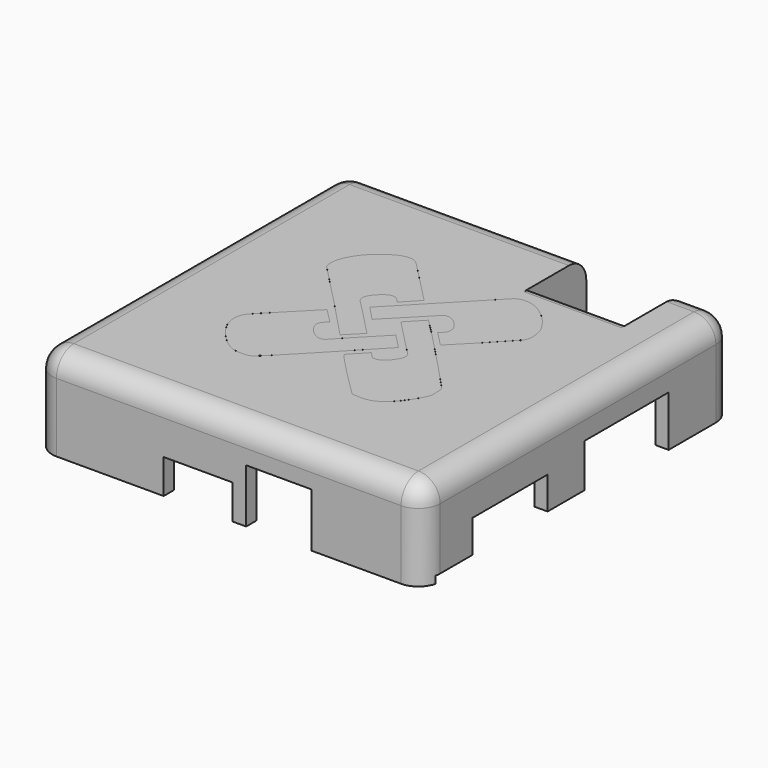
from build123d import *

# Parameters (mm, degrees)
F0_W          = 50
F0_H          = 50
F0_R          = 2.375
F1_DEPTH      = 1.5
F0_R_2        = 1.25
F2_DEPTH      = 8
F2_DEPTH_BACK = 1.5
F0_W_2        = 53.6
F0_H_2        = 53.6
F3_DEPTH      = 11
F3_DEPTH_BACK = 1.5
F4_W          = 9.5
F4_H          = 2
F4_H_2        = 2.75
F4_W_2        = 9
F4_H_3        = 2.25
F4_H_4        = 5.2
F5_DEPTH      = 26.801
F6_W          = 5.25
F6_H          = 1.1261866987
F6_W_2        = 1.14
F6_W_3        = 13
F6_H_2        = 1.5
F6_W_4        = 14.5
F6_H_3        = 6
F6_W_5        = 6.25
F6_H_4        = 3
F7_DEPTH      = 26.801
F9_W          = 9.3
F9_H          = 1.5
F9_W_2        = 1.2
F10_DEPTH     = 13.5
F11_DEPTH     = 13.5
F12_DEPTH     = 1.2
F13_T1_DEPTH  = 11.3
F13_T3_DEPTH  = 37.8
F13_T5_DEPTH  = 47.6
F13_T7_DEPTH  = 47.6
F13_T9_DEPTH  = 17
F13_T11_DEPTH = 18
F13_S15_W     = 3.06
F13_S15_H     = 3.06
F13_T16_DEPTH = 3.06
F13_S21_W     = 3.06
F13_S21_H     = 3.06
F13_T22_DEPTH = 3.06
F13_S27_W     = 3.06
F13_S27_H     = 3.06
F13_T28_DEPTH = 3.06
F13_S33_W     = 3.06
F13_S33_H     = 3.06
F13_T34_DEPTH = 3.06
F14_R         = 1.5
F15_W         = 14
F15_H         = 2
F16_DEPTH     = 26.801
F18_DEPTH     = 1.501
F19_DEPTH     = 1.5


# Not quite as in the source:
# - a fillet or chamfer that OpenCascade refuses, or shapes differently, is made with other operations: its cross-section is extruded or revolved along the edge and cut away or added


with BuildPart() as f1:
    # F0 (on Top) → F1 (new body)
    with BuildSketch(Plane.XY):
        Rectangle(F0_W, F0_H)
        with Locations((-21.5, -22)):
            Circle(F0_R, mode=Mode.SUBTRACT)
        with Locations((21.5, -22)):
            Circle(F0_R, mode=Mode.SUBTRACT)
        with Locations((-21.5, 22)):
            Circle(F0_R, mode=Mode.SUBTRACT)
        with Locations((22.25, 22)):
            Circle(F0_R, mode=Mode.SUBTRACT)
    extrude(amount=F1_DEPTH)



with BuildPart() as f1b:
    # F0 (on Top) → F1, piece 2 (new body)
    with BuildSketch(Plane.XY):
        with Locations((-21.5, 22)):
            Circle(F0_R_2)
    extrude(amount=F1_DEPTH)


with BuildPart() as f1c:
    # F0 (on Top) → F1, piece 3 (new body)
    with BuildSketch(Plane.XY):
        with Locations((22.25, 22)):
            Circle(F0_R_2)
    extrude(amount=F1_DEPTH)


with BuildPart() as f1d:
    # F0 (on Top) → F1, piece 4 (new body)
    with BuildSketch(Plane.XY):
        with Locations((21.5, -22)):
            Circle(F0_R_2)
    extrude(amount=F1_DEPTH)


with BuildPart() as f1e:
    # F0 (on Top) → F1, piece 5 (new body)
    with BuildSketch(Plane.XY):
        with Locations((-21.5, -22)):
            Circle(F0_R_2)
    extrude(amount=F1_DEPTH)


with BuildPart() as f1_1:
    add(f1.part)

    add(f1b.part)  # F2 merges F1b

    add(f1c.part)  # F2 merges F1c

    add(f1d.part)  # F2 merges F1d

    add(f1e.part)  # F2 merges F1e
    # F0 (on Top) → F2 (join, two sides)
    with BuildSketch(Plane.XY) as f2_sk:
        with Locations((-21.5, 22)):
            Circle(F0_R)
        with Locations((-21.5, 22)):
            Circle(F0_R_2, mode=Mode.SUBTRACT)
        with Locations((22.25, 22)):
            Circle(F0_R)
        with Locations((22.25, 22)):
            Circle(F0_R_2, mode=Mode.SUBTRACT)
        with Locations((21.5, -22)):
            Circle(F0_R)
        with Locations((21.5, -22)):
            Circle(F0_R_2, mode=Mode.SUBTRACT)
        with Locations((-21.5, -22)):
            Circle(F0_R)
        with Locations((-21.5, -22)):
            Circle(F0_R_2, mode=Mode.SUBTRACT)
    extrude(amount=-F2_DEPTH)
    extrude(f2_sk.sketch, amount=F2_DEPTH_BACK)

    # F0 (on Top) → F3 (join, two sides)
    with BuildSketch(Plane.XY) as f3_sk:
        Rectangle(F0_W_2, F0_H_2)
        Rectangle(F0_W, F0_H, mode=Mode.SUBTRACT)
    extrude(amount=-F3_DEPTH)
    extrude(f3_sk.sketch, amount=F3_DEPTH_BACK)

    # F4 (on Front) → F5 (cut, through all)
    with BuildSketch(Plane.XZ):
        with Locations((-4.25, -7.25)):
            Rectangle(F4_W, F4_H)
        with Locations((-4.25, -9.625)):
            Rectangle(F4_W, F4_H_2)
        with Locations((6.9, -9.875)):
            Rectangle(F4_W_2, F4_H_3)
        with Locations((6.9, -6.15)):
            Rectangle(F4_W_2, F4_H_4)
    extrude(amount=F5_DEPTH, mode=Mode.SUBTRACT)

    # F6 (on Right) → F7 (cut, through all)
    with BuildSketch(Plane.YZ):
        with Locations((-2.625, -10.5630933493)):
            Rectangle(F6_W, F6_H)
        with Locations((0.57, -10.5630933493)):
            Rectangle(F6_W_2, F6_H)
        with Locations((-11.75, -10.5630933493)):
            Rectangle(F6_W_3, F6_H)
        with Locations((-11.75, -9.25)):
            Rectangle(F6_W_3, F6_H_2)
        with Locations((8.39, -7)):
            Rectangle(F6_W_4, F6_H_3)
        with Locations((8.39, -10.5630933493)):
            Rectangle(F6_W_4, F6_H)
        with Locations((-21.375, -10.5630933493)):
            Rectangle(F6_W_5, F6_H)
        with Locations((-11.75, -7)):
            Rectangle(F6_W_3, F6_H_4)
    extrude(amount=F7_DEPTH, mode=Mode.SUBTRACT)

    # F9 (on offset) → F10 (cut)
    with BuildSketch(Plane.YZ.offset(6.5)):
        Polygon((26.8, -9), (26.8, 0), (17.5, 0), (17.5, -5.8), (17.5, -9), align=None)
        with Locations((22.15, 0.75)):
            Rectangle(F9_W, F9_H)
        Polygon((17.5, -5.8), (17.5, 0), (16.3, 0), (16.3, -9), (17.5, -9), align=None)
        with Locations((16.9, 0.75)):
            Rectangle(F9_W_2, F9_H)
    extrude(amount=F10_DEPTH, mode=Mode.SUBTRACT)

    # F9 (on offset) → F11 (join)
    with BuildSketch(Plane.YZ.offset(6.5)):
        Polygon((17.5, -5.8), (17.5, 0), (16.3, 0), (16.3, -9), (17.5, -9), align=None)
        with Locations((16.9, 0.75)):
            Rectangle(F9_W_2, F9_H)
    extrude(amount=F11_DEPTH)

    # F9 (on offset) → F12 (join)
    with BuildSketch(Plane.YZ.offset(6.5)):
        Polygon((26.8, -9), (26.8, 0), (17.5, 0), (17.5, -5.8), (17.5, -9), align=None)
        with Locations((22.15, 0.75)):
            Rectangle(F9_W, F9_H)
        Polygon((17.5, -5.8), (17.5, 0), (16.3, 0), (16.3, -9), (17.5, -9), align=None)
        with Locations((16.9, 0.75)):
            Rectangle(F9_W_2, F9_H)
    extrude(amount=-F12_DEPTH)

    # F13: fillet of radius 3 on 10 edges, made by hand

    # F13_s2 → F13_t1 (cut)
    with BuildSketch(Plane.YZ.offset(12.5)):
        with BuildLine():
            ThreePointArc((23.8, 1.5), (25.9213203436, 0.6213203436), (26.8, -1.5))
            Line((26.8, -1.5), (26.8, 1.5))
            Line((26.8, 1.5), (23.8, 1.5))
        make_face()
    extrude(amount=F13_T1_DEPTH, mode=Mode.SUBTRACT)

    # F13_s4 → F13_t3 (cut)
    with BuildSketch(Plane.YZ.offset(-23.8)):
        with BuildLine():
            ThreePointArc((23.8, 1.5), (25.9213203436, 0.6213203436), (26.8, -1.5))
            Line((26.8, -1.5), (26.8, 1.5))
            Line((26.8, 1.5), (23.8, 1.5))
        make_face()
    extrude(amount=F13_T3_DEPTH, mode=Mode.SUBTRACT)

    # F13_s6 → F13_t5 (cut)
    with BuildSketch(Plane.XZ.offset(-23.8)):
        with BuildLine():
            ThreePointArc((-23.8, 1.5), (-25.9213203436, 0.6213203436), (-26.8, -1.5))
            Line((-26.8, -1.5), (-26.8, 1.5))
            Line((-26.8, 1.5), (-23.8, 1.5))
        make_face()
        with BuildLine():
            ThreePointArc((23.8, 1.5), (25.9213203436, 0.6213203436), (26.8, -1.5))
            Line((26.8, -1.5), (26.8, 1.5))
            Line((26.8, 1.5), (23.8, 1.5))
        make_face()
    extrude(amount=F13_T5_DEPTH, mode=Mode.SUBTRACT)

    # F13_s8 → F13_t7 (cut)
    with BuildSketch(Plane.YZ.offset(-23.8)):
        with BuildLine():
            ThreePointArc((-23.8, 1.5), (-25.9213203436, 0.6213203436), (-26.8, -1.5))
            Line((-26.8, -1.5), (-26.8, 1.5))
            Line((-26.8, 1.5), (-23.8, 1.5))
        make_face()
    extrude(amount=F13_T7_DEPTH, mode=Mode.SUBTRACT)

    # F13_s10 → F13_t9 (cut)
    with BuildSketch(Plane.XY.offset(-18.5)):
        with BuildLine():
            ThreePointArc((-26.8, -23.8), (-25.9213203436, -25.9213203436), (-23.8, -26.8))
            Line((-23.8, -26.8), (-26.8, -26.8))
            Line((-26.8, -26.8), (-26.8, -23.8))
        make_face()
        with BuildLine():
            ThreePointArc((23.8, 26.8), (25.9213203436, 25.9213203436), (26.8, 23.8))
            Line((26.8, 23.8), (26.8, 26.8))
            Line((26.8, 26.8), (23.8, 26.8))
        make_face()
        with BuildLine():
            ThreePointArc((26.8, -23.8), (25.9213203436, -25.9213203436), (23.8, -26.8))
            Line((23.8, -26.8), (26.8, -26.8))
            Line((26.8, -26.8), (26.8, -23.8))
        make_face()
        with BuildLine():
            ThreePointArc((-26.8, 23.8), (-25.9213203436, 25.9213203436), (-23.8, 26.8))
            Line((-23.8, 26.8), (-26.8, 26.8))
            Line((-26.8, 26.8), (-26.8, 23.8))
        make_face()
    extrude(amount=F13_T9_DEPTH, mode=Mode.SUBTRACT)

    # F13_s12 → F13_t11 (cut)
    with BuildSketch(Plane.XY.offset(-9)):
        with BuildLine():
            ThreePointArc((23, 26.8), (20.8786796564, 25.9213203436), (20, 23.8))
            Line((20, 23.8), (20, 26.8))
            Line((20, 26.8), (23, 26.8))
        make_face()
    extrude(amount=F13_T11_DEPTH, mode=Mode.SUBTRACT)


with BuildPart() as f13_tool14:
    # F13_s15 → F13_t16 (new body)
    with BuildSketch(Plane.XY.offset(-1.5)):
        with Locations((25.33, 25.33)):
            Rectangle(F13_S15_W, F13_S15_H)
    extrude(amount=F13_T16_DEPTH)

    # F13_s17 → F13_t18 (revolve, cut)
    with BuildSketch(Plane(origin=(23.8, 23.8, -1.5), x_dir=(-0.7071067812, -0.7071067812, 0), z_dir=(-0.7071067812, 0.7071067812, 0))):
        with BuildLine():
            ThreePointArc((0, -3), (3, 0), (0, 3))
            Line((0, 3), (0, -3))
        make_face()
    revolve(axis=Axis((23.8, 23.8, -1.5), (0, 0, 1)), mode=Mode.SUBTRACT)


with BuildPart() as f1_2:
    add(f1_1.part)

    # F13_t13: cut F13_tool14
    add(f13_tool14.part, mode=Mode.SUBTRACT)


with BuildPart() as f13_tool20:
    # F13_s21 → F13_t22 (new body)
    with BuildSketch(Plane.XY.offset(-1.5)):
        with Locations((-25.33, 25.33)):
            Rectangle(F13_S21_W, F13_S21_H)
    extrude(amount=F13_T22_DEPTH)

    # F13_s23 → F13_t24 (revolve, cut)
    with BuildSketch(Plane(origin=(-23.8, 23.8, -1.5), x_dir=(0.7071067812, -0.7071067812, 0), z_dir=(-0.7071067812, -0.7071067812, 0))):
        with BuildLine():
            ThreePointArc((0, -3), (3, 0), (0, 3))
            Line((0, 3), (0, -3))
        make_face()
    revolve(axis=Axis((-23.8, 23.8, -1.5), (0, 0, 1)), mode=Mode.SUBTRACT)


with BuildPart() as f1_3:
    add(f1_2.part)

    # F13_t19: cut F13_tool20
    add(f13_tool20.part, mode=Mode.SUBTRACT)


with BuildPart() as f13_tool26:
    # F13_s27 → F13_t28 (new body)
    with BuildSketch(Plane.XY.offset(-1.5)):
        with Locations((-25.33, -25.33)):
            Rectangle(F13_S27_W, F13_S27_H)
    extrude(amount=F13_T28_DEPTH)

    # F13_s29 → F13_t30 (revolve, cut)
    with BuildSketch(Plane(origin=(-23.8, -23.8, -1.5), x_dir=(0.7071067812, 0.7071067812, 0), z_dir=(0.7071067812, -0.7071067812, 0))):
        with BuildLine():
            ThreePointArc((0, -3), (3, 0), (0, 3))
            Line((0, 3), (0, -3))
        make_face()
    revolve(axis=Axis((-23.8, -23.8, -1.5), (0, 0, 1)), mode=Mode.SUBTRACT)


with BuildPart() as f1_4:
    add(f1_3.part)

    # F13_t25: cut F13_tool26
    add(f13_tool26.part, mode=Mode.SUBTRACT)


with BuildPart() as f13_tool32:
    # F13_s33 → F13_t34 (new body)
    with BuildSketch(Plane.XY.offset(-1.5)):
        with Locations((25.33, -25.33)):
            Rectangle(F13_S33_W, F13_S33_H)
    extrude(amount=F13_T34_DEPTH)

    # F13_s35 → F13_t36 (revolve, cut)
    with BuildSketch(Plane(origin=(23.8, -23.8, -1.5), x_dir=(-0.7071067812, 0.7071067812, 0), z_dir=(0.7071067812, 0.7071067812, 0))):
        with BuildLine():
            ThreePointArc((0, -3), (3, 0), (0, 3))
            Line((0, 3), (0, -3))
        make_face()
    revolve(axis=Axis((23.8, -23.8, -1.5), (0, 0, 1)), mode=Mode.SUBTRACT)


with BuildPart() as f1_5:
    add(f1_4.part)

    # F13_t31: cut F13_tool32
    add(f13_tool32.part, mode=Mode.SUBTRACT)

    # F14
    f14_edges = [f1_5.edges().sort_by_distance(p)[0] for p in [
        (13.25, 17.5, 1.5),
    ]]
    fillet(f14_edges, radius=F14_R)

    # F15 (on Right) → F16 (cut, through all)
    with BuildSketch(Plane.YZ):
        with Locations((5.75, -7)):
            Rectangle(F15_W, F15_H)
        Polygon((0, -9), (12.75, -9), (12.75, -8), (-1.25, -8), (-1.25, -9), align=None)
        Polygon((-1.25, -10), (12.75, -10), (12.75, -9), (0, -9), (-1.25, -9), align=None)
        Polygon((24.5, -11.0357031226), (24.5, -10), (12.75, -10), (-1.25, -10), (-24.5, -10), (-24.5, -11.0357031226), align=None)
    extrude(amount=-F16_DEPTH, mode=Mode.SUBTRACT)

    # F17 (on Top) → F18 (cut, through all)
    with BuildSketch(Plane.XY):
        with BuildLine():
            add(Edge.make_bspline(
                [(2.6337690446, 4.3777345257), (4.1488296736, 2.9862137615), (13.7044419796, -7.0613876037), (13.5967130417, -7.0670198624), (13.8283273456, -7.3413269189), (13.842337494, -7.82768897), (13.8589220392, -8.8789827644), (13.8432255163, -9.4133274272), (12.1466871073, -12.5160741004), (9.4814131223, -14.6061680167), (7.0123368743, -14.178122061), (6.9283058087, -14.2847187871), (1.0148528171, -8.2934063985), (0.4936719155, -7.5717363434)],
                knots=[0.0089761431, 0.0089761431, 0.0089761431, 0.0089761431, 0.122228571, 0.1330252954, 0.1487734192, 0.1707765281, 0.2013334728, 0.2237533849, 0.2793698301, 0.3371429814, 0.3805089088, 0.3957619618, 0.4879281659, 0.4879281659, 0.4879281659, 0.4879281659], degree=3))
            Line((2.6337690446, 4.3777345257), (0.5629178592, 2.207118169))
            add(Edge.make_bspline(
                [(2.5589191396, -5.4010140019), (2.7372058883, -5.5464348869), (3.2459220871, -6.1241415889), (3.4769231626, -6.2923714077), (4.1870653829, -6.2492504655), (4.5594316814, -6.0075568322), (5.306878931, -5.4483843447), (5.7804633245, -4.6376901998), (5.9797941775, -4.3397540098), (6.0712404556, -3.8231670242), (6.0672996429, -3.3187282043), (5.1979606597, -2.5522554569), (5.2497492592, -2.6206281586), (1.2672758775, 1.4916340736), (0.5629178592, 2.207118169)],
                knots=[0.5848515334, 0.5848515334, 0.5848515334, 0.5848515334, 0.6126188416, 0.63046949, 0.6546842699, 0.6753536997, 0.7048009038, 0.7342593746, 0.752488374, 0.7735556528, 0.7960226968, 0.8266974371, 0.8357204913, 0.9100486613, 0.9100486613, 0.9100486613, 0.9100486613], degree=3))
            Line((2.5589191396, -5.4010140019), (0.4936719155, -7.5717363434))
        make_face()
        with BuildLine():
            add(Edge.make_bspline(
                [(-4.1951583095, 2.7987209668), (1.0080025634, 8.1710432624), (6.5954559155, 13.9403945733), (6.6971467282, 14.0793044814), (7.2582479051, 14.3827174509), (8.0647764726, 14.4893507471), (8.887918878, 14.3534905622), (9.7116687237, 14.0833566665), (10.7682050616, 13.4336081396), (12.09897007, 12.2967113579), (13.0658944102, 10.9673436289), (13.5917626753, 10.0740937493), (13.7533585046, 9.2948130313), (13.8487303283, 8.8038923826), (13.8752502289, 7.8516196297), (13.6781474582, 7.4110605068), (13.5859649447, 7.2050164864)],
                knots=[0.0022926657, 0.0022926657, 0.0022926657, 0.0022926657, 0.2496251328, 0.2701104018, 0.317045917, 0.3751377278, 0.4319642369, 0.4896642967, 0.5591214109, 0.6430144041, 0.7238811151, 0.7877230808, 0.8419106278, 0.8869300511, 0.9471185917, 1, 1, 1, 1], degree=3))
            Line((-4.1951583095, 2.7987209668), (-2.2396288963, 0.7255361531))
            Line((-2.2396288963, 0.7255361531), (3.0672104241, 6.1340472618))
            add(Edge.make_bspline(
                [(3.0672104241, 6.1340472618), (3.143729107, 6.2161982947), (3.297814356, 6.3859570218), (3.6778797918, 6.3840156229), (4.0031329472, 6.3985633539), (4.4692984995, 6.1750311398), (4.8561984925, 5.9176944841), (5.265564945, 5.5805325495), (5.6776892175, 5.0118322743), (6.0193058811, 4.4904086082), (5.9665132612, 3.8963677596), (6.0977186917, 3.5781533203), (5.3779196793, 2.8696377227), (5.2420848817, 2.7216840756)],
                knots=[0, 0, 0, 0, 0.0383458432, 0.0782209102, 0.1166663156, 0.1640685525, 0.2101422145, 0.2587022458, 0.3150733168, 0.3681398035, 0.4175788215, 0.4561043385, 0.5274279887, 0.5274279887, 0.5274279887, 0.5274279887], degree=3))
            Line((5.2420848817, 2.7216840756), (7.2797688511, 0.6421545641))
            add(Edge.make_bspline(
                [(7.2797688511, 0.6421545641), (7.99156258, 1.2587062345), (13.5828543825, 7.1453220507), (13.5822631613, 7.1871017459), (13.5859649447, 7.2050164864)],
                knots=[0.7622871576, 0.7622871576, 0.7622871576, 0.7622871576, 0.9617849206, 0.9820186026, 0.9820186026, 0.9820186026, 0.9820186026], degree=3))
        make_face()
        with BuildLine():
            add(Edge.make_bspline(
                [(-2.6542923727, -4.2488974646), (-2.8543834052, -4.0873226856), (-4.0845557597, -2.6800886543), (-13.7246439358, 7.2979517713), (-13.8311109945, 7.3403793646), (-13.9856307296, 7.981681817), (-13.9110669672, 9.2905656338), (-13.3101549808, 10.628786408), (-12.071793307, 12.3879190858), (-10.1704620865, 13.7773851742), (-8.9247938931, 14.4568163771), (-7.5101780435, 14.5517395208), (-6.8371715752, 14.0554988802), (-6.5565974828, 13.8000496207), (-1.1447687909, 8.2021189611), (-0.6130041743, 7.6959942927)],
                knots=[0.0720940311, 0.0720940311, 0.0720940311, 0.0720940311, 0.1166079175, 0.2264421722, 0.2371589551, 0.2589956261, 0.2931105857, 0.3289547851, 0.3725019507, 0.4179035595, 0.4534919183, 0.4877639959, 0.5119623043, 0.5362346242, 0.6202656763, 0.6202656763, 0.6202656763, 0.6202656763], degree=3))
            Line((-2.6542923727, -4.2488974646), (-0.6209075457, -2.1751756775))
            add(Edge.make_bspline(
                [(-2.62065566, 5.573224122), (-2.63628033, 5.5847033041), (-2.723374723, 5.6744621229), (-3.2713875239, 6.2899087513), (-3.6972074018, 6.4094215205), (-4.3690152372, 6.4131203892), (-5.4810347169, 5.5615218005), (-6.2571863041, 4.4573349954), (-6.2268450742, 3.4853480872), (-5.0025778643, 2.4010071339), (-2.4042081411, -0.3117811964), (-0.6209075457, -2.1751756775)],
                knots=[0.7159990353, 0.7159990353, 0.7159990353, 0.7159990353, 0.7219064655, 0.7491616781, 0.7692248412, 0.7920934858, 0.8269593183, 0.8613429851, 0.8877216064, 0.9231056494, 0.9983359861, 0.9983359861, 0.9983359861, 0.9983359861], degree=3))
            Line((-2.62065566, 5.573224122), (-0.6130041743, 7.6959942927))
        make_face()
        with BuildLine():
            add(Edge.make_bspline(
                [(4.100840015, -2.6277568325), (3.1156892088, -3.6217760081), (-6.7881001653, -14.2180707724), (-7.1441563881, -14.0552668178), (-7.6091691466, -14.2679671408), (-8.3069552716, -14.2284508947), (-9.7962702322, -14.2696213858), (-12.2148557403, -12.3291082124), (-13.9344728603, -9.855657033), (-14.1305245841, -8.0140812071), (-13.7016819828, -6.9022240008), (-13.1236888475, -6.2820192057), (-8.0022842124, -1.0662834705), (-7.4464620694, -0.530619072)],
                knots=[0.0798001793, 0.0798001793, 0.0798001793, 0.0798001793, 0.2014075833, 0.2219962522, 0.2416127947, 0.2672072339, 0.303629489, 0.3577698997, 0.4121374818, 0.4532369288, 0.4838347607, 0.5178463497, 0.6032970918, 0.6032970918, 0.6032970918, 0.6032970918], degree=3))
            Line((4.100840015, -2.6277568325), (2.0720690275, -0.5415278666))
            add(Edge.make_bspline(
                [(-5.4205875749, -2.5717176112), (-5.5411524068, -2.7060819274), (-6.3681922084, -3.4270413154), (-6.1869843049, -4.395556248), (-5.5178214749, -5.3928835237), (-4.6060598952, -6.0525376359), (-3.9678116559, -6.3417089623), (-3.2505155928, -6.148380142), (-2.6634131954, -5.3785788383), (0.0411015742, -2.6151408903), (2.0720690275, -0.5415278666)],
                knots=[0.7094889137, 0.7094889137, 0.7094889137, 0.7094889137, 0.7425186253, 0.7722751956, 0.8061471652, 0.8390403408, 0.8644863284, 0.8888753826, 0.9171555585, 0.9982612727, 0.9982612727, 0.9982612727, 0.9982612727], degree=3))
            Line((-5.4205875749, -2.5717176112), (-7.4464620694, -0.530619072))
        make_face()
    extrude(amount=F18_DEPTH, mode=Mode.SUBTRACT)


with BuildPart() as f19:
    # F17 (on Top) → F19 (new body)
    with BuildSketch(Plane.XY):
        with BuildLine():
            add(Edge.make_bspline(
                [(2.6337690446, 4.3777345257), (4.1488296736, 2.9862137615), (13.7044419796, -7.0613876037), (13.5967130417, -7.0670198624), (13.8283273456, -7.3413269189), (13.842337494, -7.82768897), (13.8589220392, -8.8789827644), (13.8432255163, -9.4133274272), (12.1466871073, -12.5160741004), (9.4814131223, -14.6061680167), (7.0123368743, -14.178122061), (6.9283058087, -14.2847187871), (1.0148528171, -8.2934063985), (0.4936719155, -7.5717363434)],
                knots=[0.0089761431, 0.0089761431, 0.0089761431, 0.0089761431, 0.122228571, 0.1330252954, 0.1487734192, 0.1707765281, 0.2013334728, 0.2237533849, 0.2793698301, 0.3371429814, 0.3805089088, 0.3957619618, 0.4879281659, 0.4879281659, 0.4879281659, 0.4879281659], degree=3))
            Line((2.6337690446, 4.3777345257), (0.5629178592, 2.207118169))
            add(Edge.make_bspline(
                [(2.5589191396, -5.4010140019), (2.7372058883, -5.5464348869), (3.2459220871, -6.1241415889), (3.4769231626, -6.2923714077), (4.1870653829, -6.2492504655), (4.5594316814, -6.0075568322), (5.306878931, -5.4483843447), (5.7804633245, -4.6376901998), (5.9797941775, -4.3397540098), (6.0712404556, -3.8231670242), (6.0672996429, -3.3187282043), (5.1979606597, -2.5522554569), (5.2497492592, -2.6206281586), (1.2672758775, 1.4916340736), (0.5629178592, 2.207118169)],
                knots=[0.5848515334, 0.5848515334, 0.5848515334, 0.5848515334, 0.6126188416, 0.63046949, 0.6546842699, 0.6753536997, 0.7048009038, 0.7342593746, 0.752488374, 0.7735556528, 0.7960226968, 0.8266974371, 0.8357204913, 0.9100486613, 0.9100486613, 0.9100486613, 0.9100486613], degree=3))
            Line((2.5589191396, -5.4010140019), (0.4936719155, -7.5717363434))
        make_face()
    extrude(amount=F19_DEPTH)


with BuildPart() as f19b:
    # F17 (on Top) → F19, piece 2 (new body)
    with BuildSketch(Plane.XY):
        with BuildLine():
            add(Edge.make_bspline(
                [(4.100840015, -2.6277568325), (3.1156892088, -3.6217760081), (-6.7881001653, -14.2180707724), (-7.1441563881, -14.0552668178), (-7.6091691466, -14.2679671408), (-8.3069552716, -14.2284508947), (-9.7962702322, -14.2696213858), (-12.2148557403, -12.3291082124), (-13.9344728603, -9.855657033), (-14.1305245841, -8.0140812071), (-13.7016819828, -6.9022240008), (-13.1236888475, -6.2820192057), (-8.0022842124, -1.0662834705), (-7.4464620694, -0.530619072)],
                knots=[0.0798001793, 0.0798001793, 0.0798001793, 0.0798001793, 0.2014075833, 0.2219962522, 0.2416127947, 0.2672072339, 0.303629489, 0.3577698997, 0.4121374818, 0.4532369288, 0.4838347607, 0.5178463497, 0.6032970918, 0.6032970918, 0.6032970918, 0.6032970918], degree=3))
            Line((4.100840015, -2.6277568325), (2.0720690275, -0.5415278666))
            add(Edge.make_bspline(
                [(-5.4205875749, -2.5717176112), (-5.5411524068, -2.7060819274), (-6.3681922084, -3.4270413154), (-6.1869843049, -4.395556248), (-5.5178214749, -5.3928835237), (-4.6060598952, -6.0525376359), (-3.9678116559, -6.3417089623), (-3.2505155928, -6.148380142), (-2.6634131954, -5.3785788383), (0.0411015742, -2.6151408903), (2.0720690275, -0.5415278666)],
                knots=[0.7094889137, 0.7094889137, 0.7094889137, 0.7094889137, 0.7425186253, 0.7722751956, 0.8061471652, 0.8390403408, 0.8644863284, 0.8888753826, 0.9171555585, 0.9982612727, 0.9982612727, 0.9982612727, 0.9982612727], degree=3))
            Line((-5.4205875749, -2.5717176112), (-7.4464620694, -0.530619072))
        make_face()
    extrude(amount=F19_DEPTH)


with BuildPart() as f19c:
    # F17 (on Top) → F19, piece 3 (new body)
    with BuildSketch(Plane.XY):
        with BuildLine():
            add(Edge.make_bspline(
                [(-2.6542923727, -4.2488974646), (-2.8543834052, -4.0873226856), (-4.0845557597, -2.6800886543), (-13.7246439358, 7.2979517713), (-13.8311109945, 7.3403793646), (-13.9856307296, 7.981681817), (-13.9110669672, 9.2905656338), (-13.3101549808, 10.628786408), (-12.071793307, 12.3879190858), (-10.1704620865, 13.7773851742), (-8.9247938931, 14.4568163771), (-7.5101780435, 14.5517395208), (-6.8371715752, 14.0554988802), (-6.5565974828, 13.8000496207), (-1.1447687909, 8.2021189611), (-0.6130041743, 7.6959942927)],
                knots=[0.0720940311, 0.0720940311, 0.0720940311, 0.0720940311, 0.1166079175, 0.2264421722, 0.2371589551, 0.2589956261, 0.2931105857, 0.3289547851, 0.3725019507, 0.4179035595, 0.4534919183, 0.4877639959, 0.5119623043, 0.5362346242, 0.6202656763, 0.6202656763, 0.6202656763, 0.6202656763], degree=3))
            Line((-2.6542923727, -4.2488974646), (-0.6209075457, -2.1751756775))
            add(Edge.make_bspline(
                [(-2.62065566, 5.573224122), (-2.63628033, 5.5847033041), (-2.723374723, 5.6744621229), (-3.2713875239, 6.2899087513), (-3.6972074018, 6.4094215205), (-4.3690152372, 6.4131203892), (-5.4810347169, 5.5615218005), (-6.2571863041, 4.4573349954), (-6.2268450742, 3.4853480872), (-5.0025778643, 2.4010071339), (-2.4042081411, -0.3117811964), (-0.6209075457, -2.1751756775)],
                knots=[0.7159990353, 0.7159990353, 0.7159990353, 0.7159990353, 0.7219064655, 0.7491616781, 0.7692248412, 0.7920934858, 0.8269593183, 0.8613429851, 0.8877216064, 0.9231056494, 0.9983359861, 0.9983359861, 0.9983359861, 0.9983359861], degree=3))
            Line((-2.62065566, 5.573224122), (-0.6130041743, 7.6959942927))
        make_face()
    extrude(amount=F19_DEPTH)


with BuildPart() as f19d:
    # F17 (on Top) → F19, piece 4 (new body)
    with BuildSketch(Plane.XY):
        with BuildLine():
            add(Edge.make_bspline(
                [(-4.1951583095, 2.7987209668), (1.0080025634, 8.1710432624), (6.5954559155, 13.9403945733), (6.6971467282, 14.0793044814), (7.2582479051, 14.3827174509), (8.0647764726, 14.4893507471), (8.887918878, 14.3534905622), (9.7116687237, 14.0833566665), (10.7682050616, 13.4336081396), (12.09897007, 12.2967113579), (13.0658944102, 10.9673436289), (13.5917626753, 10.0740937493), (13.7533585046, 9.2948130313), (13.8487303283, 8.8038923826), (13.8752502289, 7.8516196297), (13.6781474582, 7.4110605068), (13.5859649447, 7.2050164864)],
                knots=[0.0022926657, 0.0022926657, 0.0022926657, 0.0022926657, 0.2496251328, 0.2701104018, 0.317045917, 0.3751377278, 0.4319642369, 0.4896642967, 0.5591214109, 0.6430144041, 0.7238811151, 0.7877230808, 0.8419106278, 0.8869300511, 0.9471185917, 1, 1, 1, 1], degree=3))
            Line((-4.1951583095, 2.7987209668), (-2.2396288963, 0.7255361531))
            Line((-2.2396288963, 0.7255361531), (3.0672104241, 6.1340472618))
            add(Edge.make_bspline(
                [(3.0672104241, 6.1340472618), (3.143729107, 6.2161982947), (3.297814356, 6.3859570218), (3.6778797918, 6.3840156229), (4.0031329472, 6.3985633539), (4.4692984995, 6.1750311398), (4.8561984925, 5.9176944841), (5.265564945, 5.5805325495), (5.6776892175, 5.0118322743), (6.0193058811, 4.4904086082), (5.9665132612, 3.8963677596), (6.0977186917, 3.5781533203), (5.3779196793, 2.8696377227), (5.2420848817, 2.7216840756)],
                knots=[0, 0, 0, 0, 0.0383458432, 0.0782209102, 0.1166663156, 0.1640685525, 0.2101422145, 0.2587022458, 0.3150733168, 0.3681398035, 0.4175788215, 0.4561043385, 0.5274279887, 0.5274279887, 0.5274279887, 0.5274279887], degree=3))
            Line((5.2420848817, 2.7216840756), (7.2797688511, 0.6421545641))
            add(Edge.make_bspline(
                [(7.2797688511, 0.6421545641), (7.99156258, 1.2587062345), (13.5828543825, 7.1453220507), (13.5822631613, 7.1871017459), (13.5859649447, 7.2050164864)],
                knots=[0.7622871576, 0.7622871576, 0.7622871576, 0.7622871576, 0.9617849206, 0.9820186026, 0.9820186026, 0.9820186026, 0.9820186026], degree=3))
        make_face()
    extrude(amount=F19_DEPTH)


solid = Compound([f1_5.part, f19.part, f19b.part, f19c.part, f19d.part])
